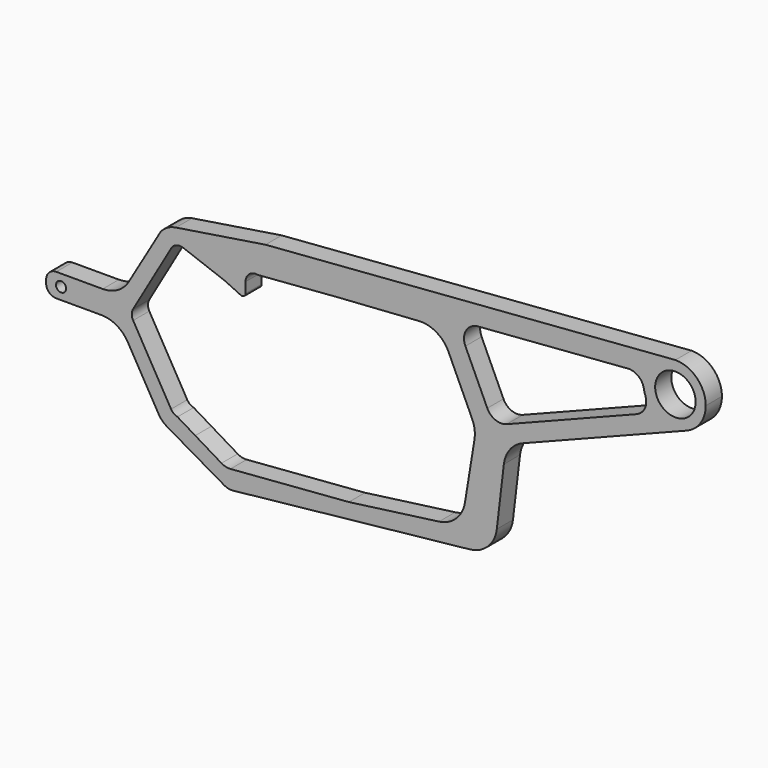
from build123d import *

# Parameters (mm, degrees)
F1_R     = 1
F1_R_2   = 4
F2_DEPTH = 4


# Not quite as in the source:
# - a feature names something its author has since deleted; it is built from what else it names


with BuildPart() as f2:
    # F1 (on Front) → F2 (new body)
    with BuildSketch(Plane.XZ):
        with BuildLine():
            ThreePointArc((53.6725900561, -3.4803708923), (56.4360817028, -1.2749098512), (57.4778270766, 2.1038045583))
            ThreePointArc((57.4778270766, 2.1038045583), (55.7204672392, 6.3464457699), (51.4778255932, 8.1038045583))
            Line((51.4778255932, 8.1038045583), (-29.5767494715, 1.8164854333))
            Line((-29.5767494715, 1.8164854333), (-47.2952228074, -0.9563085456))
            ThreePointArc((-47.2952228074, -0.9563085456), (-48.9181443858, -1.5076422035), (-50.2595064205, -2.5746900675))
            Line((-50.2595064205, -2.5746900675), (-56.5978536574, -13.3921147633))
            ThreePointArc((-56.5978536574, -13.3921147633), (-58.7913353541, -15.5645829823), (-61.7746472195, -16.3588313254))
            Line((-61.7746472195, -16.3588313254), (-70.9623719458, -16.3588313254))
            ThreePointArc((-70.9623719458, -16.3588313254), (-72.3660357626, -16.9341461359), (-72.9621509967, -18.3291034361))
            Line((-72.9621509967, -18.3291034361), (-72.9714351561, -18.9536438246))
            ThreePointArc((-72.9714351561, -18.9536438246), (-72.3963412947, -20.3870355307), (-70.9716561052, -20.9833717139))
            Line((-70.9716561052, -20.9833717139), (-62.0211355409, -20.9833717139))
            ThreePointArc((-62.0211355409, -20.9833717139), (-59.0238889239, -21.7856305971), (-56.8281648814, -23.977867475))
            Line((-56.8281648814, -23.977867475), (-51.1217613336, -33.8375062708))
            Line((-51.1217613336, -33.8375062708), (-50.5134866975, -34.8884954183))
            ThreePointArc((-50.5134866975, -34.8884954183), (-49.834113752, -35.622752626), (-49.0221729234, -36.2070755993))
            Line((-49.0221729234, -36.2070755993), (-37.7895467449, -42.6922353472))
            ThreePointArc((-37.7895467449, -42.6922353472), (-36.9110233024, -43.029081092), (-35.9713694581, -43.0772386209))
            Line((-35.9713694581, -43.0772386209), (10.8377953956, -38.0845412605))
            ThreePointArc((10.8377953956, -38.0845412605), (14.4191592098, -36.3857997297), (16.1597362046, -32.824580657))
            Line((16.1597362046, -32.824580657), (17.5522645357, -21.0756224064))
            ThreePointArc((17.5522645357, -21.0756224064), (18.760112016, -18.1166816586), (21.3157969388, -16.1976453223))
            Line((21.3157969388, -16.1976453223), (53.6725900561, -3.4803708923))
        make_face()
        with Locations((-70.0084173118, -18.6587822488)):
            Circle(F1_R, mode=Mode.SUBTRACT)
        with BuildLine():
            ThreePointArc((-33.5221489054, -5.8863848639), (-32.7820426942, -4.3428905644), (-31.1190403454, -3.9372367165))
            Line((-31.1190403454, -3.9372367165), (-15.3857114758, -2.6969403245))
            ThreePointArc((-15.3857114758, -2.6969403245), (-15.3533597704, -2.6945658839), (-15.320984282, -2.6925413929))
            Line((-15.320984282, -2.6925413929), (0.7603415418, -1.5996367209))
            ThreePointArc((0.7603415418, -1.5996367209), (4.2304854801, -2.4267493449), (6.6177460931, -5.0775984562))
            Line((6.6177460931, -5.0775984562), (11.2725159026, -15.1927708333))
            ThreePointArc((11.2725159026, -15.1927708333), (11.7672314644, -16.8926047847), (11.7443467828, -18.6628181167))
            Line((11.7443467828, -18.6628181167), (9.8637327358, -30.2427322728))
            ThreePointArc((9.8637327358, -30.2427322728), (8.1254532697, -33.5812724587), (4.7405491326, -35.2274468291))
            Line((4.7405491326, -35.2274468291), (-13.1016644536, -37.6254695609))
            Line((-13.1016644536, -37.6254695609), (-36.5010263621, -39.4700978904))
            ThreePointArc((-36.5010263621, -39.4700978904), (-37.4240833549, -39.3995872417), (-38.2816944982, -39.0510057009))
            Line((-38.2816944982, -39.0510057009), (-43.475593846, -35.9307785793))
            Line((-43.475593846, -35.9307785793), (-46.9845830439, -33.8227586638))
            ThreePointArc((-46.9845830439, -33.8227586638), (-47.7169758073, -33.480833261), (-48.2542237632, -32.8769485246))
            Line((-48.2542237632, -32.8769485246), (-55.7535278454, -19.8877718654))
            ThreePointArc((-55.7535278454, -19.8877718654), (-56.0221729234, -18.8865675237), (-55.7535278454, -17.8853631819))
            Line((-55.7535278454, -17.8853631819), (-48.3466238348, -5.0768093424))
            ThreePointArc((-48.3466238348, -5.0768093424), (-47.2942991525, -4.0512417288), (-45.8251853322, -4.0215642922))
            Line((-45.8251853322, -4.0215642922), (-37.9265817129, -6.9582780391))
            Line((-37.9265817129, -6.9582780391), (-37.6259790546, -7.0700425992))
            Line((-37.6259790546, -7.0700425992), (-34.4656276648, -8.5558833842))
            ThreePointArc((-34.4656276648, -8.5558833842), (-33.8292769309, -8.5156852397), (-33.5221489054, -7.9569093245))
            Line((-33.5221489054, -7.9569093245), (-33.5221489054, -5.9059880699))
            ThreePointArc((-33.5221489054, -5.9059880699), (-33.5221729234, -5.8961864669), (-33.5221489054, -5.8863848639))
        make_face(mode=Mode.SUBTRACT)
        with BuildLine():
            ThreePointArc((9.9534750477, -2.9862699605), (10.0919340096, -0.2128411234), (12.4467532901, 1.2588601217))
            Line((12.4467532901, 1.2588601217), (42.0606238873, 3.555977278))
            ThreePointArc((42.0606238873, 3.555977278), (44.1407275048, 2.9281273611), (45.2513978552, 1.0606590347))
            ThreePointArc((45.2513978552, 1.0606590347), (45.3681686541, 0.5136324312), (45.5329001833, -0.0209113441))
            ThreePointArc((45.5329001833, -0.0209113441), (45.4391256015, -2.2717054042), (43.8052859559, -3.8226520781))
            Line((43.8052859559, -3.8226520781), (18.1020868014, -13.9248471934))
            ThreePointArc((18.1020868014, -13.9248471934), (15.884946368, -13.9159482702), (14.2794171364, -12.3868744398))
            Line((14.2794171364, -12.3868744398), (9.9534750477, -2.9862699605))
        make_face(mode=Mode.SUBTRACT)
        with Locations((51.4778270766, 2.1038045583)):
            Circle(F1_R_2, mode=Mode.SUBTRACT)
    extrude(amount=F2_DEPTH)


solid = f2.part
